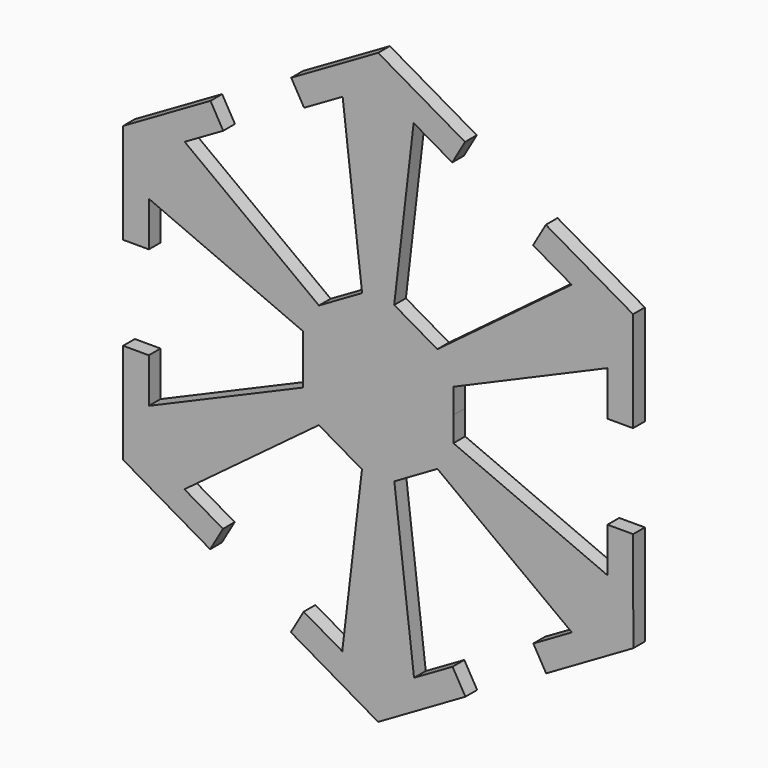
from build123d import *

# Parameters (mm, degrees)
F1_DEPTH = 1.27


# Not quite as in the source:
# - ends of sketch curves that miss each other by under 0.0002 mm in the source are joined


with BuildPart() as f1:
    # F0 (on Front) → F1 (new body)
    with BuildSketch(Plane.XZ):
        Polygon((-44.6418710053, 40.8897735178), (-44.6418710053, 33.3539977979), (-44.6297971524, 33.3609944811), (-43.2404409197, 34.166113231), (-39.5050764062, 36.3307215128), (-38.1157201735, 37.1358402628), (-38.1182953477, 38.7416174302), (-38.1217403313, 40.8897735313), (-38.1217487156, 40.8950016529), align=None)
        Polygon((-44.6539448582, 33.3609944811), (-44.6418710053, 33.3539977979), (-44.6418710053, 40.8897735178), (-51.161993295, 40.8950016529), (-51.161993295, 40.8897735178), (-51.1654466629, 38.7416174302), (-51.1680218371, 37.1358402628), (-49.7786656044, 36.3307215128), (-46.0433010909, 34.166113231), align=None)
        Polygon((-44.6418710053, 40.8897735178), (-38.1217487156, 40.8950016529), (-38.1217487156, 40.9002297812), (-38.1217487156, 43.0483886446), (-38.1217487156, 44.6541678769), (-39.5123943237, 45.4570574931), (-43.2512253972, 47.6156726199), (-44.6418710053, 48.418562236), align=None)
        Polygon((-51.161993295, 40.8950016529), (-44.6418710053, 40.8897735178), (-44.6418710053, 48.418562236), (-46.0325166134, 47.6156726199), (-49.7713476869, 45.4570574931), (-51.161993295, 44.6541678769), (-51.161993295, 43.0483886446), (-51.161993295, 40.9002297812), align=None)
        Polygon((-41.5661535928, 62.0498394063), (-44.6418710053, 63.8223188678), (-44.6418710053, 48.418562236), (-43.2512253972, 47.6156726199), align=None)
        Polygon((-44.6418710053, 48.418562236), (-44.6418710053, 63.8223188678), (-47.7175884178, 62.0498394063), (-46.0325166134, 47.6156726199), align=None)
        Polygon((-37.1105166727, 62.0498394063), (-44.6418710053, 66.3980688576), (-44.6418710053, 63.8223188678), (-41.5661535928, 62.0498394063), (-38.2213332575, 60.1222808724), align=None)
        Polygon((-44.6418710053, 63.8223188678), (-44.6418710053, 66.3980688576), (-52.1732253379, 62.0498394063), (-51.0624087531, 60.1222808724), (-47.7175884178, 62.0498394063), align=None)
        Polygon((-24.7788576939, 48.806157048), (-24.7757621839, 44.9456783996), (-22.5510392338, 44.9474622851), (-22.5510392338, 53.6439211877), (-30.1115337683, 58.0089747424), (-31.2206558067, 56.0879190201), (-27.8758354714, 54.1603604862), (-24.7817211845, 52.3772792439), align=None)
        Polygon((-38.1217487156, 43.0483886446), (-24.7788576939, 48.806157048), (-24.7817211845, 52.3772792439), (-27.8758354714, 54.1603604862), (-39.5123943237, 45.4570574931), (-38.1217487156, 44.6541678769), align=None)
        Polygon((-22.5445603606, 36.8675168429), (-24.7692833106, 36.8657329574), (-24.7661878006, 33.0052543089), (-24.76332431, 29.4341321131), (-27.8545751064, 27.6460911595), (-31.1962999317, 25.713171045), (-30.0840985392, 23.7938964823), (-22.5306139252, 28.1710691232), align=None)
        Polygon((-24.76332431, 29.4341321131), (-24.7661878006, 33.0052543089), (-38.1182953477, 38.7416174302), (-38.1157201735, 37.1358402628), (-39.5050764062, 36.3307215128), (-27.8545751064, 27.6460911595), align=None)
        Polygon((-44.6827784364, 15.3815109795), (-44.6418710053, 15.3578055115), (-44.6418710053, 33.3539977979), (-44.6539448582, 33.3609944811), (-46.0433010909, 34.166113231), (-47.7515186761, 19.7346673406), (-51.0932435014, 21.6675874551), (-52.2071498666, 19.7418128067), align=None)
        Polygon((-44.6418710053, 33.3539977979), (-44.6418710053, 15.3578055115), (-44.6009635742, 15.3815109795), (-37.076592144, 19.7418128067), (-38.1904985092, 21.6675874551), (-41.5322233345, 19.7346673406), (-43.2404409197, 34.166113231), (-44.6297971524, 33.3609944811), align=None)
        Polygon((-51.1654466629, 38.7416174302), (-64.5175542099, 33.0052543089), (-64.5204177006, 29.4341321131), (-61.4291669042, 27.6460911595), (-49.7786656044, 36.3307215128), (-51.1680218371, 37.1358402628), align=None)
        Polygon((-64.5144587, 36.8657329574), (-66.73918165, 36.8675168429), (-66.7531280854, 28.1710691232), (-59.1996434714, 23.7938964823), (-58.0874420789, 25.713171045), (-61.4291669042, 27.6460911595), (-64.5204177006, 29.4341321131), (-64.5175542099, 33.0052543089), align=None)
        Polygon((-64.5020208261, 52.3772792439), (-64.5048843167, 48.806157048), (-51.161993295, 43.0483886446), (-51.161993295, 44.6541678769), (-49.7713476869, 45.4570574931), (-61.4079065392, 54.1603604862), align=None)
        Polygon((-58.0630862039, 56.0879190201), (-59.1722082423, 58.0089747424), (-66.7327027768, 53.6439211877), (-66.7327027768, 44.9474622851), (-64.5079798267, 44.9456783996), (-64.5048843167, 48.806157048), (-64.5020208261, 52.3772792439), (-61.4079065392, 54.1603604862), align=None)
    extrude(amount=F1_DEPTH)


solid = f1.part
